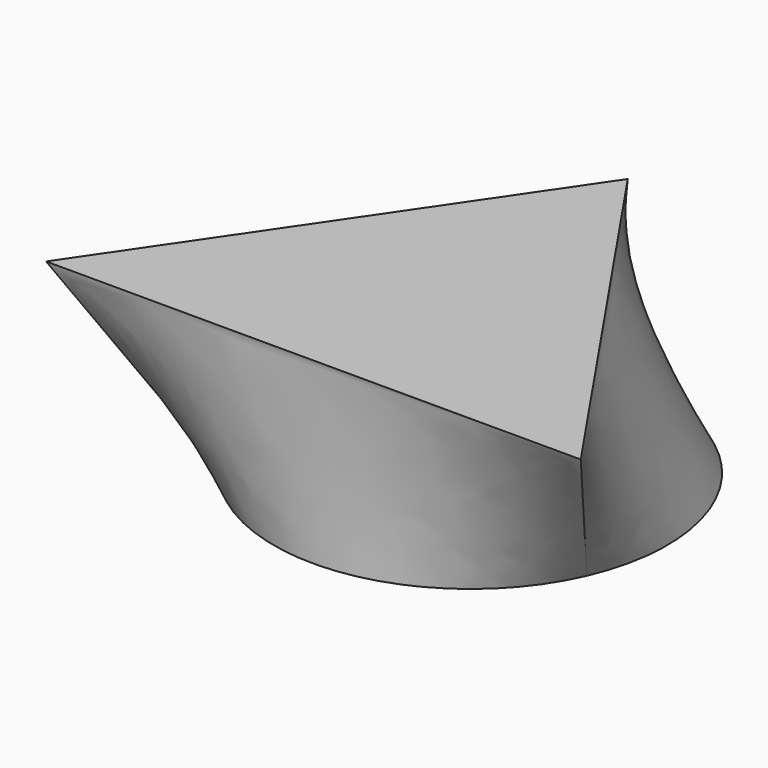
from build123d import *


# Not quite as in the source:
# - the arcs of a loft's sections are written as splines that run evenly, so that the points pair up as in the source's solid


with BuildPart() as f3:
    # F2 (on offset) → F3 section 0
    with BuildSketch(Plane.XY.offset(50.8)):
        Polygon((0, 55.9030920267), (-76.0614573956, -55.6952729821), (76.0614573956, -55.9030920267), align=None)
    # F0 (on Top) → F3 section 1
    with BuildSketch(Plane.XY):
        with BuildLine():
            add(Edge.make_bspline(
                [(-45.0678651205, -33.0005121721), (-43.1479731463, -35.6224542827), (-40.9987241522, -38.0763897141), (-36.3066842111, -42.5738360658), (-33.7639657227, -44.6172775328), (-28.3622350481, -48.2316333835), (-25.5033062801, -49.8024919512), (-19.5560137252, -52.4239369272), (-16.4677417815, -53.4744828529), (-10.155592821, -55.0233656751), (-6.931813282, -55.5216786525), (-0.446599368, -55.9509373002), (2.8147348565, -55.8818763415), (9.2759637808, -55.1784680079), (12.4757587007, -54.5441314956), (18.716681464, -52.7294288869), (21.7577129298, -51.5490908148), (27.5887022521, -48.6782327515), (30.3785700614, -46.9877570947), (35.6224542827, -43.1479731463), (38.0763897141, -40.9987241522), (42.5738360658, -36.3066842111), (44.6172775328, -33.7639657227), (48.2316333835, -28.3622350481), (49.8024919512, -25.5033062801), (51.1132144392, -22.5296600026)],
                knots=[0, 0, 0, 0, 0.0833333333, 0.0833333333, 0.1666666667, 0.1666666667, 0.25, 0.25, 0.3333333333, 0.3333333333, 0.4166666667, 0.4166666667, 0.5, 0.5, 0.5833333333, 0.5833333333, 0.6666666667, 0.6666666667, 0.75, 0.75, 0.8333333333, 0.8333333333, 0.9166666667, 0.9166666667, 1, 1, 1, 1], degree=3))
            add(Edge.make_bspline(
                [(51.1132144392, -22.5296600026), (52.4239369272, -19.5560137252), (53.4744828529, -16.4677417815), (55.0233656751, -10.155592821), (55.5216786525, -6.931813282), (55.9509373002, -0.446599368), (55.8818763415, 2.8147348565), (55.1784680079, 9.2759637808), (54.5441314956, 12.4757587007), (52.7294288869, 18.716681464), (51.5490908148, 21.7577129298), (48.6782327515, 27.5887022521), (46.9877570947, 30.3785700614), (43.1479731463, 35.6224542827), (40.9987241522, 38.0763897141), (36.3066842111, 42.5738360658), (33.7639657227, 44.6172775328), (28.3622350481, 48.2316333835), (25.5033062801, 49.8024919512), (19.5560137252, 52.4239369272), (16.4677417815, 53.4744828529), (10.155592821, 55.0233656751), (6.931813282, 55.5216786525), (0.446599368, 55.9509373002), (-2.8147348565, 55.8818763415), (-6.0453493187, 55.5301721747)],
                knots=[0, 0, 0, 0, 0.0833333333, 0.0833333333, 0.1666666667, 0.1666666667, 0.25, 0.25, 0.3333333333, 0.3333333333, 0.4166666667, 0.4166666667, 0.5, 0.5, 0.5833333333, 0.5833333333, 0.6666666667, 0.6666666667, 0.75, 0.75, 0.8333333333, 0.8333333333, 0.9166666667, 0.9166666667, 1, 1, 1, 1], degree=3))
            add(Edge.make_bspline(
                [(-6.0453493187, 55.5301721747), (-9.2759637808, 55.1784680079), (-12.4757587007, 54.5441314956), (-18.716681464, 52.7294288869), (-21.7577129298, 51.5490908148), (-27.5887022521, 48.6782327515), (-30.3785700614, 46.9877570947), (-35.6224542827, 43.1479731463), (-38.0763897141, 40.9987241522), (-42.5738360658, 36.3066842111), (-44.6172775328, 33.7639657227), (-48.2316333835, 28.3622350481), (-49.8024919512, 25.5033062801), (-52.4239369272, 19.5560137252), (-53.4744828529, 16.4677417815), (-55.0233656751, 10.155592821), (-55.5216786525, 6.931813282), (-55.9509373002, 0.446599368), (-55.8818763415, -2.8147348565), (-55.1784680079, -9.2759637808), (-54.5441314956, -12.4757587007), (-52.7294288869, -18.716681464), (-51.5490908148, -21.7577129298), (-48.6782327515, -27.5887022521), (-46.9877570947, -30.3785700614), (-45.0678651205, -33.0005121721)],
                knots=[0, 0, 0, 0, 0.0833333333, 0.0833333333, 0.1666666667, 0.1666666667, 0.25, 0.25, 0.3333333333, 0.3333333333, 0.4166666667, 0.4166666667, 0.5, 0.5, 0.5833333333, 0.5833333333, 0.6666666667, 0.6666666667, 0.75, 0.75, 0.8333333333, 0.8333333333, 0.9166666667, 0.9166666667, 1, 1, 1, 1], degree=3))
        make_face()
    loft(ruled=True)


solid = f3.part
